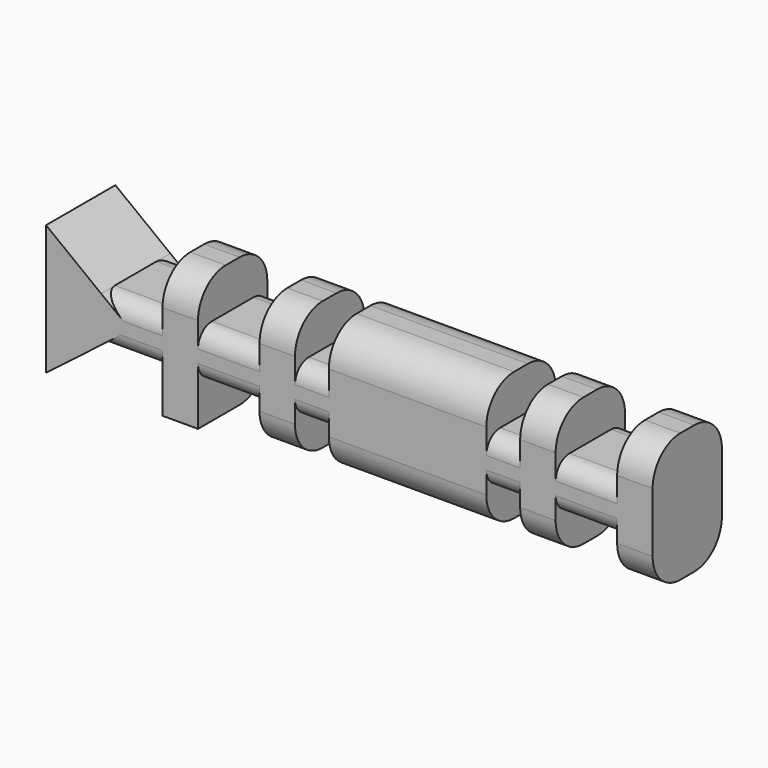
from build123d import *

# Parameters (mm, degrees)
F0_W          = 18.0351980008
F0_H          = 13.9310602441
F0_W_2        = 9.9258822108
F1_DEPTH      = 25.4
F2_R          = 10.16
F3_T1_DEPTH   = 18.0351980008
F3_T3_DEPTH   = 9.9258822108
F3_T5_DEPTH   = 18.0351980008
F3_T7_DEPTH   = 9.9258822108
F3_T12_DEPTH  = 43.4351980008
F3_T17_DEPTH  = 30.7351980008
F3_T22_DEPTH  = 30.7351980008
F3_T27_DEPTH  = 43.4351980008
F3_T32_DEPTH  = 43.4351980008
F3_T37_DEPTH  = 30.7351980008
F3_T42_DEPTH  = 30.7351980008
F3_T47_DEPTH  = 43.4351980008
F3_T52_DEPTH  = 43.4351980008
F3_T57_DEPTH  = 43.4351980008
F3_T62_DEPTH  = 43.4351980008
F3_T67_DEPTH  = 43.4351980008
F3_T72_DEPTH  = 43.4351980008
F3_T77_DEPTH  = 43.4351980008
F3_T82_DEPTH  = 43.4351980008
F3_T87_DEPTH  = 43.4351980008
F3_T92_DEPTH  = 35.3258822108
F3_T97_DEPTH  = 35.3258822108
F3_T102_DEPTH = 35.3258822108
F3_T107_DEPTH = 35.3258822108
F3_T112_DEPTH = 43.4351980008
F3_T117_DEPTH = 43.4351980008
F3_T122_DEPTH = 43.4351980008
F3_T127_DEPTH = 43.4351980008
F3_T132_DEPTH = 35.3258822108
F3_T137_DEPTH = 35.3258822108
F3_T142_DEPTH = 35.3258822108
F3_T147_DEPTH = 35.3258822108


# Not quite as in the source:
# - a fillet or chamfer that OpenCascade refuses, or shapes differently, is made with other operations: its cross-section is extruded or revolved along the edge and cut away or added


with BuildPart() as f1:
    # F0 (on Front) → F1 (new body)
    with BuildSketch(Plane.XZ):
        Polygon((-60.7531283318, 6.7454743419), (-76.858874061, 19.1352828354), (-76.858874061, -18.9647171646), (-60.7531283318, -6.5749086711), align=None)
        Polygon((-42.717930331, 6.7454743419), (-60.7531283318, 6.7454743419), (-60.7531283318, -6.5749086711), (-60.7531283318, -7.1855859023), (-42.717930331, -7.1855859023), align=None)
        Polygon((-42.717930331, 19.1352828354), (-42.717930331, 6.7454743419), (-42.717930331, -7.1855859023), (-42.717930331, -18.9647171646), (-32.3238125419, -18.9647171646), (-32.3238125419, -7.1855859023), (-32.3238125419, 6.7454743419), (-32.3238125419, 19.1352828354), align=None)
        with Locations((-23.3062135415, -0.2200557802)):
            Rectangle(F0_W, F0_H)
        Polygon((-14.2886145411, 19.1352828354), (-14.2886145411, 6.7454743419), (-14.2886145411, -7.1855859023), (-14.2886145411, -18.6845511312), (-3.8944967519, -18.6845511312), (-3.8944967519, -7.1855859023), (-3.8944967519, 6.7454743419), (-3.8944967519, 19.1352828354), align=None)
        with Locations((1.0684443535, -0.2200557802)):
            Rectangle(F0_W_2, F0_H)
        Polygon((6.0313854589, 19.1352828354), (6.0313854589, 6.7454743419), (6.0313854589, -7.1855859023), (6.0313854589, -18.6845511312), (52.191810149, -18.6845511312), (52.191810149, -7.1855859023), (52.191810149, 6.7454743419), (52.191810149, 19.1352828354), align=None)
        with Locations((57.1547512544, -0.2200557802)):
            Rectangle(F0_W_2, F0_H)
        Polygon((62.1176923599, 19.1352828354), (62.1176923599, 6.7454743419), (62.1176923599, -7.1855859023), (62.1176923599, -18.6845511312), (72.511810149, -18.6845511312), (72.511810149, -7.1855859023), (72.511810149, 6.7454743419), (72.511810149, 19.1352828354), align=None)
        with Locations((81.5294091494, -0.2200557802)):
            Rectangle(F0_W, F0_H)
        Polygon((90.5470081498, 19.1352828354), (90.5470081498, 6.7454743419), (90.5470081498, -7.1855859023), (90.5470081498, -18.6845511312), (100.941125939, -18.6845511312), (100.941125939, 19.1352828354), align=None)
    extrude(amount=F1_DEPTH)

    # F2
    f2_edges = [f1.edges().sort_by_distance(p)[0] for p in [
        (67.314751, 0, -18.684551),
        (67.314751, -25.4, -18.684551),
        (95.744067, 0, -18.684551),
        (95.744067, -25.4, -18.684551),
        (95.744067, -25.4, 19.135283),
        (95.744067, 0, 19.135283),
        (67.314751, -25.4, 19.135283),
        (67.314751, 0, 19.135283),
        (29.111598, -25.4, 19.135283),
        (29.111598, 0, 19.135283),
        (29.111598, -25.4, -18.684551),
        (29.111598, 0, -18.684551),
        (-9.091556, 0, 19.135283),
        (-9.091556, 0, -18.684551),
        (-9.091556, -25.4, 19.135283),
        (-9.091556, -25.4, -18.684551),
        (-37.520871, 0, 19.135283),
        (-37.520871, 0, -18.964717),
        (-37.520871, -25.4, 19.135283),
    ]]
    fillet(f2_edges, radius=F2_R)

    # F3: fillet of radius 5.08 on 20 edges, made by hand

    # F3_s2 → F3_t1 (cut)
    with BuildSketch(Plane.YZ.offset(-32.3238125419)):
        with BuildLine():
            ThreePointArc((0, 1.6654743419), (-1.4878975516, 5.2575767903), (-5.08, 6.7454743419))
            Line((-5.08, 6.7454743419), (0, 6.7454743419))
            Line((0, 6.7454743419), (0, 1.6654743419))
        make_face()
        with BuildLine():
            ThreePointArc((0, -2.1055859023), (-1.4878975516, -5.6976883507), (-5.08, -7.1855859023))
            Line((-5.08, -7.1855859023), (0, -7.1855859023))
            Line((0, -7.1855859023), (0, -2.1055859023))
        make_face()
        with BuildLine():
            ThreePointArc((-25.4, 1.6654743419), (-23.9121024484, 5.2575767903), (-20.32, 6.7454743419))
            Line((-20.32, 6.7454743419), (-25.4, 6.7454743419))
            Line((-25.4, 6.7454743419), (-25.4, 1.6654743419))
        make_face()
        with BuildLine():
            ThreePointArc((-25.4, -2.1055859023), (-23.9121024484, -5.6976883507), (-20.32, -7.1855859023))
            Line((-20.32, -7.1855859023), (-25.4, -7.1855859023))
            Line((-25.4, -7.1855859023), (-25.4, -2.1055859023))
        make_face()
    extrude(amount=F3_T1_DEPTH, mode=Mode.SUBTRACT)

    # F3_s4 → F3_t3 (cut)
    with BuildSketch(Plane.YZ.offset(-3.8944967519)):
        with BuildLine():
            ThreePointArc((-25.4, 1.6654743419), (-23.9121024484, 5.2575767903), (-20.32, 6.7454743419))
            Line((-20.32, 6.7454743419), (-25.4, 6.7454743419))
            Line((-25.4, 6.7454743419), (-25.4, 1.6654743419))
        make_face()
        with BuildLine():
            ThreePointArc((-25.4, -2.1055859023), (-23.9121024484, -5.6976883507), (-20.32, -7.1855859023))
            Line((-20.32, -7.1855859023), (-25.4, -7.1855859023))
            Line((-25.4, -7.1855859023), (-25.4, -2.1055859023))
        make_face()
        with BuildLine():
            ThreePointArc((0, 1.6654743419), (-1.4878975516, 5.2575767903), (-5.08, 6.7454743419))
            Line((-5.08, 6.7454743419), (0, 6.7454743419))
            Line((0, 6.7454743419), (0, 1.6654743419))
        make_face()
        with BuildLine():
            ThreePointArc((0, -2.1055859023), (-1.4878975516, -5.6976883507), (-5.08, -7.1855859023))
            Line((-5.08, -7.1855859023), (0, -7.1855859023))
            Line((0, -7.1855859023), (0, -2.1055859023))
        make_face()
    extrude(amount=F3_T3_DEPTH, mode=Mode.SUBTRACT)

    # F3_s6 → F3_t5 (cut)
    with BuildSketch(Plane.YZ.offset(72.511810149)):
        with BuildLine():
            ThreePointArc((0, 1.6654743419), (-1.4878975516, 5.2575767903), (-5.08, 6.7454743419))
            Line((-5.08, 6.7454743419), (0, 6.7454743419))
            Line((0, 6.7454743419), (0, 1.6654743419))
        make_face()
        with BuildLine():
            ThreePointArc((-25.4, 1.6654743419), (-23.9121024484, 5.2575767903), (-20.32, 6.7454743419))
            Line((-20.32, 6.7454743419), (-25.4, 6.7454743419))
            Line((-25.4, 6.7454743419), (-25.4, 1.6654743419))
        make_face()
        with BuildLine():
            ThreePointArc((-25.4, -2.1055859023), (-23.9121024484, -5.6976883507), (-20.32, -7.1855859023))
            Line((-20.32, -7.1855859023), (-25.4, -7.1855859023))
            Line((-25.4, -7.1855859023), (-25.4, -2.1055859023))
        make_face()
        with BuildLine():
            ThreePointArc((0, -2.1055859023), (-1.4878975516, -5.6976883507), (-5.08, -7.1855859023))
            Line((-5.08, -7.1855859023), (0, -7.1855859023))
            Line((0, -7.1855859023), (0, -2.1055859023))
        make_face()
    extrude(amount=F3_T5_DEPTH, mode=Mode.SUBTRACT)

    # F3_s8 → F3_t7 (cut)
    with BuildSketch(Plane.YZ.offset(52.191810149)):
        with BuildLine():
            ThreePointArc((0, 1.6654743419), (-1.4878975516, 5.2575767903), (-5.08, 6.7454743419))
            Line((-5.08, 6.7454743419), (0, 6.7454743419))
            Line((0, 6.7454743419), (0, 1.6654743419))
        make_face()
        with BuildLine():
            ThreePointArc((-25.4, 1.6654743419), (-23.9121024484, 5.2575767903), (-20.32, 6.7454743419))
            Line((-20.32, 6.7454743419), (-25.4, 6.7454743419))
            Line((-25.4, 6.7454743419), (-25.4, 1.6654743419))
        make_face()
        with BuildLine():
            ThreePointArc((0, -2.1055859023), (-1.4878975516, -5.6976883507), (-5.08, -7.1855859023))
            Line((-5.08, -7.1855859023), (0, -7.1855859023))
            Line((0, -7.1855859023), (0, -2.1055859023))
        make_face()
        with BuildLine():
            ThreePointArc((-25.4, -2.1055859023), (-23.9121024484, -5.6976883507), (-20.32, -7.1855859023))
            Line((-20.32, -7.1855859023), (-25.4, -7.1855859023))
            Line((-25.4, -7.1855859023), (-25.4, -2.1055859023))
        make_face()
    extrude(amount=F3_T7_DEPTH, mode=Mode.SUBTRACT)


with BuildPart() as f3_tool10:
    # F3_s11 → F3_t12 (new body)
    with BuildSketch(Plane.YZ.offset(-30.017930331)):
        with BuildLine():
            ThreePointArc((-25.4, 1.6654743419), (-23.9121024484, 5.2575767903), (-20.32, 6.7454743419))
            Line((-20.32, 6.7454743419), (-25.4, 6.7454743419))
            Line((-25.4, 6.7454743419), (-25.4, 1.6654743419))
        make_face()
    extrude(amount=-F3_T12_DEPTH)

    split(bisect_by=Plane.YZ.offset(-32.3238125419), keep=Keep.TOP)


with BuildPart() as f1_1:
    add(f1.part)

    # F3_t9: cut F3_tool10
    add(f3_tool10.part, mode=Mode.SUBTRACT)


with BuildPart() as f3_tool15:
    # F3_s16 → F3_t17 (new body)
    with BuildSketch(Plane.YZ.offset(-42.717930331)):
        with BuildLine():
            ThreePointArc((-25.4, 1.6654743419), (-23.9121024484, 5.2575767903), (-20.32, 6.7454743419))
            Line((-20.32, 6.7454743419), (-25.4, 6.7454743419))
            Line((-25.4, 6.7454743419), (-25.4, 1.6654743419))
        make_face()
    extrude(amount=-F3_T17_DEPTH)

    split(bisect_by=Plane(origin=(-19.3266305302, 0, -25.1230515214), x_dir=(0, 1, 0), z_dir=(0.60973467, 0, 0.7926055969)), keep=Keep.TOP)


with BuildPart() as f1_2:
    add(f1_1.part)

    # F3_t14: cut F3_tool15
    add(f3_tool15.part, mode=Mode.SUBTRACT)


with BuildPart() as f3_tool20:
    # F3_s21 → F3_t22 (new body)
    with BuildSketch(Plane.YZ.offset(-73.4531283318)):
        with BuildLine():
            ThreePointArc((-25.4, -2.1055859023), (-23.9121024484, -5.6976883507), (-20.32, -7.1855859023))
            Line((-20.32, -7.1855859023), (-25.4, -7.1855859023))
            Line((-25.4, -7.1855859023), (-25.4, -2.1055859023))
        make_face()
    extrude(amount=F3_T22_DEPTH)

    split(bisect_by=Plane(origin=(-19.4090613561, 0, 25.2302049066), x_dir=(0, 1, 0), z_dir=(0.60973467, 0, -0.7926055969)), keep=Keep.TOP)


with BuildPart() as f1_3:
    add(f1_2.part)

    # F3_t19: cut F3_tool20
    add(f3_tool20.part, mode=Mode.SUBTRACT)


with BuildPart() as f3_tool25:
    # F3_s26 → F3_t27 (new body)
    with BuildSketch(Plane.YZ.offset(-73.4531283318)):
        with BuildLine():
            ThreePointArc((-25.4, -2.1055859023), (-23.9121024484, -5.6976883507), (-20.32, -7.1855859023))
            Line((-20.32, -7.1855859023), (-25.4, -7.1855859023))
            Line((-25.4, -7.1855859023), (-25.4, -2.1055859023))
        make_face()
    extrude(amount=F3_T27_DEPTH)

    split(bisect_by=Plane.YZ.offset(-32.3238125419), keep=Keep.TOP)


with BuildPart() as f1_4:
    add(f1_3.part)

    # F3_t24: cut F3_tool25
    add(f3_tool25.part, mode=Mode.SUBTRACT)


with BuildPart() as f3_tool30:
    # F3_s31 → F3_t32 (new body)
    with BuildSketch(Plane.YZ.offset(-30.017930331)):
        with BuildLine():
            ThreePointArc((0, 1.6654743419), (-1.4878975516, 5.2575767903), (-5.08, 6.7454743419))
            Line((-5.08, 6.7454743419), (0, 6.7454743419))
            Line((0, 6.7454743419), (0, 1.6654743419))
        make_face()
    extrude(amount=-F3_T32_DEPTH)

    split(bisect_by=Plane.YZ.offset(-32.3238125419), keep=Keep.TOP)


with BuildPart() as f1_5:
    add(f1_4.part)

    # F3_t29: cut F3_tool30
    add(f3_tool30.part, mode=Mode.SUBTRACT)


with BuildPart() as f3_tool35:
    # F3_s36 → F3_t37 (new body)
    with BuildSketch(Plane.YZ.offset(-42.717930331)):
        with BuildLine():
            ThreePointArc((0, 1.6654743419), (-1.4878975516, 5.2575767903), (-5.08, 6.7454743419))
            Line((-5.08, 6.7454743419), (0, 6.7454743419))
            Line((0, 6.7454743419), (0, 1.6654743419))
        make_face()
    extrude(amount=-F3_T37_DEPTH)

    split(bisect_by=Plane(origin=(-19.3266305302, 0, -25.1230515214), x_dir=(0, 1, 0), z_dir=(0.60973467, 0, 0.7926055969)), keep=Keep.TOP)


with BuildPart() as f1_6:
    add(f1_5.part)

    # F3_t34: cut F3_tool35
    add(f3_tool35.part, mode=Mode.SUBTRACT)


with BuildPart() as f3_tool40:
    # F3_s41 → F3_t42 (new body)
    with BuildSketch(Plane.YZ.offset(-73.4531283318)):
        with BuildLine():
            ThreePointArc((0, -2.1055859023), (-1.4878975516, -5.6976883507), (-5.08, -7.1855859023))
            Line((-5.08, -7.1855859023), (0, -7.1855859023))
            Line((0, -7.1855859023), (0, -2.1055859023))
        make_face()
    extrude(amount=F3_T42_DEPTH)

    split(bisect_by=Plane(origin=(-19.4090613561, 0, 25.2302049066), x_dir=(0, 1, 0), z_dir=(0.60973467, 0, -0.7926055969)), keep=Keep.TOP)


with BuildPart() as f1_7:
    add(f1_6.part)

    # F3_t39: cut F3_tool40
    add(f3_tool40.part, mode=Mode.SUBTRACT)


with BuildPart() as f3_tool45:
    # F3_s46 → F3_t47 (new body)
    with BuildSketch(Plane.YZ.offset(-73.4531283318)):
        with BuildLine():
            ThreePointArc((0, -2.1055859023), (-1.4878975516, -5.6976883507), (-5.08, -7.1855859023))
            Line((-5.08, -7.1855859023), (0, -7.1855859023))
            Line((0, -7.1855859023), (0, -2.1055859023))
        make_face()
    extrude(amount=F3_T47_DEPTH)

    split(bisect_by=Plane.YZ.offset(-32.3238125419), keep=Keep.TOP)


with BuildPart() as f1_8:
    add(f1_7.part)

    # F3_t44: cut F3_tool45
    add(f3_tool45.part, mode=Mode.SUBTRACT)


with BuildPart() as f3_tool50:
    # F3_s51 → F3_t52 (new body)
    with BuildSketch(Plane.YZ.offset(-1.5886145411)):
        with BuildLine():
            ThreePointArc((0, 1.6654743419), (-1.4878975516, 5.2575767903), (-5.08, 6.7454743419))
            Line((-5.08, 6.7454743419), (0, 6.7454743419))
            Line((0, 6.7454743419), (0, 1.6654743419))
        make_face()
    extrude(amount=-F3_T52_DEPTH)

    split(bisect_by=Plane.YZ.offset(-3.8944967519), keep=Keep.TOP)


with BuildPart() as f1_9:
    add(f1_8.part)

    # F3_t49: cut F3_tool50
    add(f3_tool50.part, mode=Mode.SUBTRACT)


with BuildPart() as f3_tool55:
    # F3_s56 → F3_t57 (new body)
    with BuildSketch(Plane.YZ.offset(-1.5886145411)):
        with BuildLine():
            ThreePointArc((0, 1.6654743419), (-1.4878975516, 5.2575767903), (-5.08, 6.7454743419))
            Line((-5.08, 6.7454743419), (0, 6.7454743419))
            Line((0, 6.7454743419), (0, 1.6654743419))
        make_face()
    extrude(amount=-F3_T57_DEPTH)

    split(bisect_by=Plane.YZ.offset(-42.717930331), keep=Keep.BOTTOM)


with BuildPart() as f1_10:
    add(f1_9.part)

    # F3_t54: cut F3_tool55
    add(f3_tool55.part, mode=Mode.SUBTRACT)


with BuildPart() as f3_tool60:
    # F3_s61 → F3_t62 (new body)
    with BuildSketch(Plane.YZ.offset(-45.0238125419)):
        with BuildLine():
            ThreePointArc((0, -2.1055859023), (-1.4878975516, -5.6976883507), (-5.08, -7.1855859023))
            Line((-5.08, -7.1855859023), (0, -7.1855859023))
            Line((0, -7.1855859023), (0, -2.1055859023))
        make_face()
    extrude(amount=F3_T62_DEPTH)

    split(bisect_by=Plane.YZ.offset(-42.717930331), keep=Keep.BOTTOM)


with BuildPart() as f1_11:
    add(f1_10.part)

    # F3_t59: cut F3_tool60
    add(f3_tool60.part, mode=Mode.SUBTRACT)


with BuildPart() as f3_tool65:
    # F3_s66 → F3_t67 (new body)
    with BuildSketch(Plane.YZ.offset(-45.0238125419)):
        with BuildLine():
            ThreePointArc((0, -2.1055859023), (-1.4878975516, -5.6976883507), (-5.08, -7.1855859023))
            Line((-5.08, -7.1855859023), (0, -7.1855859023))
            Line((0, -7.1855859023), (0, -2.1055859023))
        make_face()
    extrude(amount=F3_T67_DEPTH)

    split(bisect_by=Plane.YZ.offset(-3.8944967519), keep=Keep.TOP)


with BuildPart() as f1_12:
    add(f1_11.part)

    # F3_t64: cut F3_tool65
    add(f3_tool65.part, mode=Mode.SUBTRACT)


with BuildPart() as f3_tool70:
    # F3_s71 → F3_t72 (new body)
    with BuildSketch(Plane.YZ.offset(-1.5886145411)):
        with BuildLine():
            ThreePointArc((-25.4, 1.6654743419), (-23.9121024484, 5.2575767903), (-20.32, 6.7454743419))
            Line((-20.32, 6.7454743419), (-25.4, 6.7454743419))
            Line((-25.4, 6.7454743419), (-25.4, 1.6654743419))
        make_face()
    extrude(amount=-F3_T72_DEPTH)

    split(bisect_by=Plane.YZ.offset(-3.8944967519), keep=Keep.TOP)


with BuildPart() as f1_13:
    add(f1_12.part)

    # F3_t69: cut F3_tool70
    add(f3_tool70.part, mode=Mode.SUBTRACT)


with BuildPart() as f3_tool75:
    # F3_s76 → F3_t77 (new body)
    with BuildSketch(Plane.YZ.offset(-1.5886145411)):
        with BuildLine():
            ThreePointArc((-25.4, 1.6654743419), (-23.9121024484, 5.2575767903), (-20.32, 6.7454743419))
            Line((-20.32, 6.7454743419), (-25.4, 6.7454743419))
            Line((-25.4, 6.7454743419), (-25.4, 1.6654743419))
        make_face()
    extrude(amount=-F3_T77_DEPTH)

    split(bisect_by=Plane.YZ.offset(-42.717930331), keep=Keep.BOTTOM)


with BuildPart() as f1_14:
    add(f1_13.part)

    # F3_t74: cut F3_tool75
    add(f3_tool75.part, mode=Mode.SUBTRACT)


with BuildPart() as f3_tool80:
    # F3_s81 → F3_t82 (new body)
    with BuildSketch(Plane.YZ.offset(-45.0238125419)):
        with BuildLine():
            ThreePointArc((-25.4, -2.1055859023), (-23.9121024484, -5.6976883507), (-20.32, -7.1855859023))
            Line((-20.32, -7.1855859023), (-25.4, -7.1855859023))
            Line((-25.4, -7.1855859023), (-25.4, -2.1055859023))
        make_face()
    extrude(amount=F3_T82_DEPTH)

    split(bisect_by=Plane.YZ.offset(-42.717930331), keep=Keep.BOTTOM)


with BuildPart() as f1_15:
    add(f1_14.part)

    # F3_t79: cut F3_tool80
    add(f3_tool80.part, mode=Mode.SUBTRACT)


with BuildPart() as f3_tool85:
    # F3_s86 → F3_t87 (new body)
    with BuildSketch(Plane.YZ.offset(-45.0238125419)):
        with BuildLine():
            ThreePointArc((-25.4, -2.1055859023), (-23.9121024484, -5.6976883507), (-20.32, -7.1855859023))
            Line((-20.32, -7.1855859023), (-25.4, -7.1855859023))
            Line((-25.4, -7.1855859023), (-25.4, -2.1055859023))
        make_face()
    extrude(amount=F3_T87_DEPTH)

    split(bisect_by=Plane.YZ.offset(-3.8944967519), keep=Keep.TOP)


with BuildPart() as f1_16:
    add(f1_15.part)

    # F3_t84: cut F3_tool85
    add(f3_tool85.part, mode=Mode.SUBTRACT)


with BuildPart() as f3_tool90:
    # F3_s91 → F3_t92 (new body)
    with BuildSketch(Plane.YZ.offset(18.7313854589)):
        with BuildLine():
            ThreePointArc((-25.4, 1.6654743419), (-23.9121024484, 5.2575767903), (-20.32, 6.7454743419))
            Line((-20.32, 6.7454743419), (-25.4, 6.7454743419))
            Line((-25.4, 6.7454743419), (-25.4, 1.6654743419))
        make_face()
    extrude(amount=-F3_T92_DEPTH)

    split(bisect_by=Plane.YZ.offset(-14.2886145411), keep=Keep.BOTTOM)


with BuildPart() as f1_17:
    add(f1_16.part)

    # F3_t89: cut F3_tool90
    add(f3_tool90.part, mode=Mode.SUBTRACT)


with BuildPart() as f3_tool95:
    # F3_s96 → F3_t97 (new body)
    with BuildSketch(Plane.YZ.offset(-16.5944967519)):
        with BuildLine():
            ThreePointArc((-25.4, -2.1055859023), (-23.9121024484, -5.6976883507), (-20.32, -7.1855859023))
            Line((-20.32, -7.1855859023), (-25.4, -7.1855859023))
            Line((-25.4, -7.1855859023), (-25.4, -2.1055859023))
        make_face()
    extrude(amount=F3_T97_DEPTH)

    split(bisect_by=Plane.YZ.offset(-14.2886145411), keep=Keep.BOTTOM)


with BuildPart() as f1_18:
    add(f1_17.part)

    # F3_t94: cut F3_tool95
    add(f3_tool95.part, mode=Mode.SUBTRACT)


with BuildPart() as f3_tool100:
    # F3_s101 → F3_t102 (new body)
    with BuildSketch(Plane.YZ.offset(18.7313854589)):
        with BuildLine():
            ThreePointArc((0, 1.6654743419), (-1.4878975516, 5.2575767903), (-5.08, 6.7454743419))
            Line((-5.08, 6.7454743419), (0, 6.7454743419))
            Line((0, 6.7454743419), (0, 1.6654743419))
        make_face()
    extrude(amount=-F3_T102_DEPTH)

    split(bisect_by=Plane.YZ.offset(-14.2886145411), keep=Keep.BOTTOM)


with BuildPart() as f1_19:
    add(f1_18.part)

    # F3_t99: cut F3_tool100
    add(f3_tool100.part, mode=Mode.SUBTRACT)


with BuildPart() as f3_tool105:
    # F3_s106 → F3_t107 (new body)
    with BuildSketch(Plane.YZ.offset(-16.5944967519)):
        with BuildLine():
            ThreePointArc((0, -2.1055859023), (-1.4878975516, -5.6976883507), (-5.08, -7.1855859023))
            Line((-5.08, -7.1855859023), (0, -7.1855859023))
            Line((0, -7.1855859023), (0, -2.1055859023))
        make_face()
    extrude(amount=F3_T107_DEPTH)

    split(bisect_by=Plane.YZ.offset(-14.2886145411), keep=Keep.BOTTOM)


with BuildPart() as f1_20:
    add(f1_19.part)

    # F3_t104: cut F3_tool105
    add(f3_tool105.part, mode=Mode.SUBTRACT)


with BuildPart() as f3_tool110:
    # F3_s111 → F3_t112 (new body)
    with BuildSketch(Plane.YZ.offset(103.2470081498)):
        with BuildLine():
            ThreePointArc((0, 1.6654743419), (-1.4878975516, 5.2575767903), (-5.08, 6.7454743419))
            Line((-5.08, 6.7454743419), (0, 6.7454743419))
            Line((0, 6.7454743419), (0, 1.6654743419))
        make_face()
    extrude(amount=-F3_T112_DEPTH)

    split(bisect_by=Plane.YZ.offset(62.1176923599), keep=Keep.BOTTOM)


with BuildPart() as f1_21:
    add(f1_20.part)

    # F3_t109: cut F3_tool110
    add(f3_tool110.part, mode=Mode.SUBTRACT)


with BuildPart() as f3_tool115:
    # F3_s116 → F3_t117 (new body)
    with BuildSketch(Plane.YZ.offset(103.2470081498)):
        with BuildLine():
            ThreePointArc((-25.4, 1.6654743419), (-23.9121024484, 5.2575767903), (-20.32, 6.7454743419))
            Line((-20.32, 6.7454743419), (-25.4, 6.7454743419))
            Line((-25.4, 6.7454743419), (-25.4, 1.6654743419))
        make_face()
    extrude(amount=-F3_T117_DEPTH)

    split(bisect_by=Plane.YZ.offset(62.1176923599), keep=Keep.BOTTOM)


with BuildPart() as f1_22:
    add(f1_21.part)

    # F3_t114: cut F3_tool115
    add(f3_tool115.part, mode=Mode.SUBTRACT)


with BuildPart() as f3_tool120:
    # F3_s121 → F3_t122 (new body)
    with BuildSketch(Plane.YZ.offset(59.811810149)):
        with BuildLine():
            ThreePointArc((-25.4, -2.1055859023), (-23.9121024484, -5.6976883507), (-20.32, -7.1855859023))
            Line((-20.32, -7.1855859023), (-25.4, -7.1855859023))
            Line((-25.4, -7.1855859023), (-25.4, -2.1055859023))
        make_face()
    extrude(amount=F3_T122_DEPTH)

    split(bisect_by=Plane.YZ.offset(62.1176923599), keep=Keep.BOTTOM)


with BuildPart() as f1_23:
    add(f1_22.part)

    # F3_t119: cut F3_tool120
    add(f3_tool120.part, mode=Mode.SUBTRACT)


with BuildPart() as f3_tool125:
    # F3_s126 → F3_t127 (new body)
    with BuildSketch(Plane.YZ.offset(59.811810149)):
        with BuildLine():
            ThreePointArc((0, -2.1055859023), (-1.4878975516, -5.6976883507), (-5.08, -7.1855859023))
            Line((-5.08, -7.1855859023), (0, -7.1855859023))
            Line((0, -7.1855859023), (0, -2.1055859023))
        make_face()
    extrude(amount=F3_T127_DEPTH)

    split(bisect_by=Plane.YZ.offset(62.1176923599), keep=Keep.BOTTOM)


with BuildPart() as f1_24:
    add(f1_23.part)

    # F3_t124: cut F3_tool125
    add(f3_tool125.part, mode=Mode.SUBTRACT)


with BuildPart() as f3_tool130:
    # F3_s131 → F3_t132 (new body)
    with BuildSketch(Plane.YZ.offset(74.8176923599)):
        with BuildLine():
            ThreePointArc((0, 1.6654743419), (-1.4878975516, 5.2575767903), (-5.08, 6.7454743419))
            Line((-5.08, 6.7454743419), (0, 6.7454743419))
            Line((0, 6.7454743419), (0, 1.6654743419))
        make_face()
    extrude(amount=-F3_T132_DEPTH)

    split(bisect_by=Plane.YZ.offset(72.511810149), keep=Keep.TOP)


with BuildPart() as f1_25:
    add(f1_24.part)

    # F3_t129: cut F3_tool130
    add(f3_tool130.part, mode=Mode.SUBTRACT)


with BuildPart() as f3_tool135:
    # F3_s136 → F3_t137 (new body)
    with BuildSketch(Plane.YZ.offset(74.8176923599)):
        with BuildLine():
            ThreePointArc((-25.4, 1.6654743419), (-23.9121024484, 5.2575767903), (-20.32, 6.7454743419))
            Line((-20.32, 6.7454743419), (-25.4, 6.7454743419))
            Line((-25.4, 6.7454743419), (-25.4, 1.6654743419))
        make_face()
    extrude(amount=-F3_T137_DEPTH)

    split(bisect_by=Plane.YZ.offset(72.511810149), keep=Keep.TOP)


with BuildPart() as f1_26:
    add(f1_25.part)

    # F3_t134: cut F3_tool135
    add(f3_tool135.part, mode=Mode.SUBTRACT)


with BuildPart() as f3_tool140:
    # F3_s141 → F3_t142 (new body)
    with BuildSketch(Plane.YZ.offset(39.491810149)):
        with BuildLine():
            ThreePointArc((0, -2.1055859023), (-1.4878975516, -5.6976883507), (-5.08, -7.1855859023))
            Line((-5.08, -7.1855859023), (0, -7.1855859023))
            Line((0, -7.1855859023), (0, -2.1055859023))
        make_face()
    extrude(amount=F3_T142_DEPTH)

    split(bisect_by=Plane.YZ.offset(72.511810149), keep=Keep.TOP)


with BuildPart() as f1_27:
    add(f1_26.part)

    # F3_t139: cut F3_tool140
    add(f3_tool140.part, mode=Mode.SUBTRACT)


with BuildPart() as f3_tool145:
    # F3_s146 → F3_t147 (new body)
    with BuildSketch(Plane.YZ.offset(39.491810149)):
        with BuildLine():
            ThreePointArc((-25.4, -2.1055859023), (-23.9121024484, -5.6976883507), (-20.32, -7.1855859023))
            Line((-20.32, -7.1855859023), (-25.4, -7.1855859023))
            Line((-25.4, -7.1855859023), (-25.4, -2.1055859023))
        make_face()
    extrude(amount=F3_T147_DEPTH)

    split(bisect_by=Plane.YZ.offset(72.511810149), keep=Keep.TOP)


with BuildPart() as f1_28:
    add(f1_27.part)

    # F3_t144: cut F3_tool145
    add(f3_tool145.part, mode=Mode.SUBTRACT)


solid = f1_28.part
